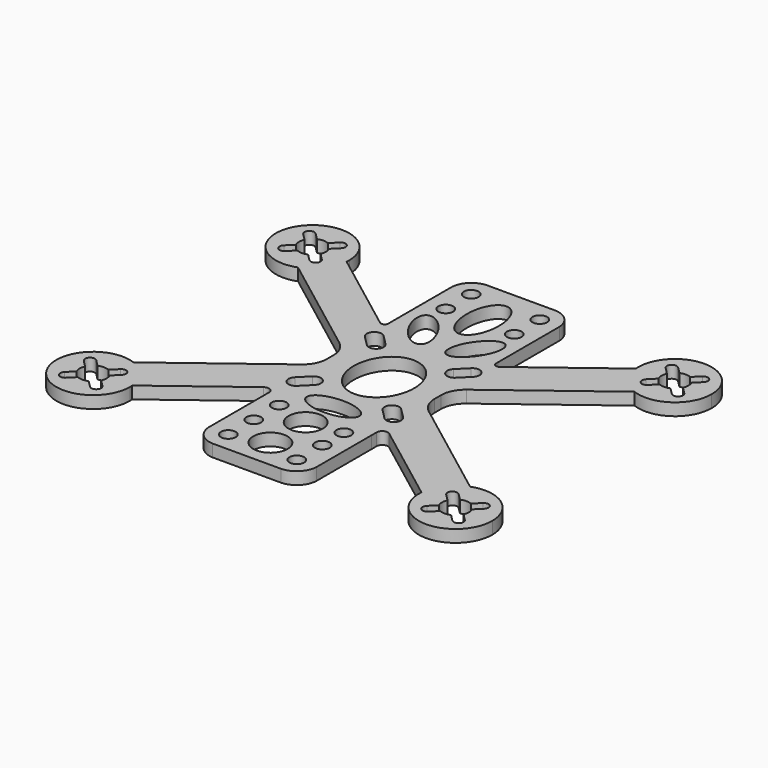
from build123d import *

# Parameters (mm, degrees)
F0_R     = 1.5
F0_R_2   = 3.5
F1_DEPTH = 2.5


# Not quite as in the source:
# - ends of sketch curves that miss each other by under 0.0002 mm in the source are joined


with BuildPart() as f1:
    # F0 (on Top) → F1 (new body)
    with BuildSketch(Plane.XY):
        with BuildLine():
            ThreePointArc((34.3547960707, 20.9819592355), (41.2667886361, 21.831976432), (44.5, 28))
            ThreePointArc((44.5, 28), (36.6803140057, 35.4931836268), (29.5272531026, 27.3612091045))
            ThreePointArc((29.5272531026, 27.3612091045), (31.0194532478, 23.4741784675), (34.3547960707, 20.9819592355))
        make_face()
        with BuildLine():
            ThreePointArc((39.5185288745, 29.1043153121), (39.6915102085, 28.5641567137), (39.75, 28))
            ThreePointArc((39.75, 28), (39.6915102085, 27.4358432863), (39.5185288745, 26.8956846879))
            Line((39.5185288745, 26.8956846879), (40.8890872965, 25.5251262658))
            ThreePointArc((40.8890872965, 25.5251262658), (41.1058600479, 25.200702917), (41.1819805153, 24.8180194847))
            ThreePointArc((41.1819805153, 24.8180194847), (40.5646639477, 23.8941399521), (39.4748737342, 24.1109127035))
            Line((39.4748737342, 24.1109127035), (38.1043153121, 25.4814711255))
            ThreePointArc((38.1043153121, 25.4814711255), (37, 25.25), (35.8956846879, 25.4814711255))
            Line((35.8956846879, 25.4814711255), (34.5251262658, 24.1109127035))
            ThreePointArc((34.5251262658, 24.1109127035), (33.1109127035, 24.1109127035), (33.1109127035, 25.5251262658))
            Line((33.1109127035, 25.5251262658), (34.4814711255, 26.8956846879))
            ThreePointArc((34.4814711255, 26.8956846879), (34.25, 28), (34.4814711255, 29.1043153121))
            Line((34.4814711255, 29.1043153121), (33.1109127035, 30.4748737342))
            ThreePointArc((33.1109127035, 30.4748737342), (33.1109127035, 31.8890872965), (34.5251262659, 31.8890872965))
            Line((34.5251262659, 31.8890872965), (35.8956846879, 30.5185288745))
            ThreePointArc((35.8956846879, 30.5185288745), (37, 30.75), (38.1043153121, 30.5185288745))
            Line((38.1043153121, 30.5185288745), (39.4748737342, 31.8890872965))
            ThreePointArc((39.4748737342, 31.8890872965), (40.5646639477, 32.1058600479), (41.1819805153, 31.1819805153))
            ThreePointArc((41.1819805153, 31.1819805153), (41.1058600479, 30.799297083), (40.8890872965, 30.4748737342))
            Line((40.8890872965, 30.4748737342), (39.5185288745, 29.1043153121))
        make_face(mode=Mode.SUBTRACT)
        with BuildLine():
            ThreePointArc((34.3547960707, 20.9819592355), (31.0194532478, 23.4741784675), (29.5272531026, 27.3612091045))
            Line((29.5272531026, 27.3612091045), (12.1863106506, 14.2383327238))
            ThreePointArc((12.1863106506, 14.2383327238), (11.4103948027, 14.1658389401), (10.9999810531, 14.8283050191))
            Line((10.9999810531, 14.8283050191), (10.9999810531, 15.3887438851))
            Line((10.9999810531, 15.3887438851), (11, 30.9999999999))
            ThreePointArc((11, 30.9999999999), (9.7793705992, 33.7793705992), (7, 35))
            Line((7, 35), (-7, 35))
            ThreePointArc((-7, 35), (-9.7793705992, 33.7793705992), (-11, 30.9999999999))
            Line((-11, 30.9999999999), (-11.0000189469, 15.3887625552))
            Line((-11.0000189469, 15.3887625552), (-11.0000085785, 14.8283395373))
            ThreePointArc((-11.0000085785, 14.8283395373), (-11.4104161998, 14.1658628176), (-12.1863381759, 14.2383535537))
            Line((-12.1863381759, 14.2383535537), (-29.5272531027, 27.3612091045))
            ThreePointArc((-29.5272531027, 27.3612091045), (-31.0194532478, 23.4741784675), (-34.3547960707, 20.9819592355))
            Line((-34.3547960707, 20.9819592355), (-12.9827933492, 4.8085505238))
            ThreePointArc((-12.9827933492, 4.8085505238), (-11.5230630838, 3.0479451115), (-11.0000068481, 0.8215228605))
            Line((-11.0000068481, 0.8215228605), (-11.0000054834, -0.8215135223))
            ThreePointArc((-11.0000054834, -0.8215135223), (-11.52305987, -3.0479403605), (-12.9827919846, -4.8085494911))
            Line((-12.9827919846, -4.8085494911), (-34.3547960707, -20.9819592355))
            ThreePointArc((-34.3547960707, -20.9819592355), (-31.0194532478, -23.4741784675), (-29.5272531026, -27.3612091045))
            Line((-29.5272531026, -27.3612091045), (-12.8232836871, -14.7203664102))
            ThreePointArc((-12.8232836871, -14.7203664102), (-11.6307646479, -14.6089516643), (-10.9999982035, -15.6271110806))
            Line((-10.9999982035, -15.6271110806), (-11.0000078854, -16.9179276686))
            Line((-11.0000078854, -16.9179276686), (-11, -30.9999999999))
            ThreePointArc((-11, -30.9999999999), (-9.7793705992, -33.7793705992), (-7, -35))
            Line((-7, -35), (7, -35))
            ThreePointArc((7, -35), (9.7793705992, -33.7793705992), (11, -30.9999999999))
            Line((11, -30.9999999999), (11.0000078854, -16.9179276686))
            Line((11.0000078854, -16.9179276686), (10.9999982035, -15.6271110806))
            ThreePointArc((10.9999982035, -15.6271110806), (11.6307646479, -14.6089516643), (12.8232836871, -14.7203664102))
            Line((12.8232836871, -14.7203664102), (29.5272531027, -27.3612091045))
            ThreePointArc((29.5272531027, -27.3612091045), (31.0194532478, -23.4741784675), (34.3547960707, -20.9819592355))
            Line((34.3547960707, -20.9819592355), (12.9827810177, -4.8085411919))
            ThreePointArc((12.9827810177, -4.8085411919), (11.5230507523, -3.0479357796), (10.9999945166, -0.8215135285))
            Line((10.9999945166, -0.8215135285), (10.999993152, 0.8215041904))
            ThreePointArc((10.999993152, 0.8215041904), (11.5230475385, 3.0479310286), (12.9827796531, 4.8085401592))
            Line((12.9827796531, 4.8085401592), (34.3547960707, 20.9819592355))
        make_face()
        with Locations((-7, -30.9999999999)):
            Circle(F0_R, mode=Mode.SUBTRACT)
        with Locations((-7, -24.4999999999)):
            Circle(F0_R, mode=Mode.SUBTRACT)
        with Locations((-7, -17.9999999999)):
            Circle(F0_R, mode=Mode.SUBTRACT)
        with BuildLine():
            ThreePointArc((-9.0606601718, -6.9393398282), (-7.4259748515, -6.6141807012), (-6.5, -8))
            ThreePointArc((-6.5, -8), (-6.6141807012, -8.5740251485), (-6.9393398282, -9.0606601717))
            Line((-6.9393398282, -9.0606601717), (-8.9393398282, -11.0606601717))
            ThreePointArc((-8.9393398282, -11.0606601717), (-11.0606601718, -11.0606601718), (-11.0606601718, -8.9393398282))
            Line((-11.0606601718, -8.9393398282), (-9.0606601718, -6.9393398282))
        make_face(mode=Mode.SUBTRACT)
        with Locations((0, -28.9999999999)):
            Circle(F0_R_2, mode=Mode.SUBTRACT)
        with Locations((7, -30.9999999999)):
            Circle(F0_R, mode=Mode.SUBTRACT)
        with Locations((7, -24.5)):
            Circle(F0_R, mode=Mode.SUBTRACT)
        with Locations((0, -19.9999999999)):
            Circle(F0_R_2, mode=Mode.SUBTRACT)
        with Locations((7, -19)):
            Circle(F0_R, mode=Mode.SUBTRACT)
        with BuildLine():
            add(Edge.make_bspline(
                [(5.3534731269, -12.9912551492), (5.3534731269, -8.6611281303), (-2.6767365634, -10.8261916398), (-10.7069462538, -12.9912551492), (-2.6767365634, -15.1563186587), (5.3534731269, -17.3213821682), (5.3534731269, -12.9912551492)],
                knots=[0, 0, 0, 2.0943951024, 2.0943951024, 4.1887902048, 4.1887902048, 6.2831853072, 6.2831853072, 6.2831853072], degree=2, weights=[1, 0.5, 1, 0.5, 1, 0.5, 1]))
        make_face(mode=Mode.SUBTRACT)
        with BuildLine():
            ThreePointArc((6.9393398282, -9.0606601717), (6.9393398282, -6.9393398282), (9.0606601718, -6.9393398282))
            Line((9.0606601718, -6.9393398282), (11.0606601718, -8.9393398282))
            ThreePointArc((11.0606601718, -8.9393398282), (11.3858192988, -9.4259748515), (11.5, -10))
            ThreePointArc((11.5, -10), (10.5740251485, -11.3858192988), (8.9393398282, -11.0606601717))
            Line((8.9393398282, -11.0606601717), (6.9393398282, -9.0606601717))
        make_face(mode=Mode.SUBTRACT)
        with BuildLine():
            ThreePointArc((-6.9393398282, 9.0606601717), (-6.6141807012, 8.5740251485), (-6.5, 8))
            ThreePointArc((-6.5, 8), (-7.4259748515, 6.6141807012), (-9.0606601718, 6.9393398282))
            Line((-9.0606601718, 6.9393398282), (-11.0606601718, 8.9393398282))
            ThreePointArc((-11.0606601718, 8.9393398282), (-11.0606601718, 11.0606601718), (-8.9393398282, 11.0606601717))
            Line((-8.9393398282, 11.0606601717), (-6.9393398282, 9.0606601717))
        make_face(mode=Mode.SUBTRACT)
        with BuildLine():
            add(Edge.make_bspline(
                [(-2.6455968618, 12.4099850655), (0.8605262478, 14.6258535456), (-4.929215171, 19.9050748086), (-10.7189565897, 25.1842960715), (-8.4353382806, 17.6892063284), (-6.1517199715, 10.1941165853), (-2.6455968618, 12.4099850655)],
                knots=[0, 0, 0, 2.0943951024, 2.0943951024, 4.1887902048, 4.1887902048, 6.2831853072, 6.2831853072, 6.2831853072], degree=2, weights=[1, 0.5, 1, 0.5, 1, 0.5, 1]))
        make_face(mode=Mode.SUBTRACT)
        with Locations((-7, 24.4999999999)):
            Circle(F0_R, mode=Mode.SUBTRACT)
        with Locations((-7, 30.9999999999)):
            Circle(F0_R, mode=Mode.SUBTRACT)
        with BuildLine():
            add(Edge.make_bspline(
                [(6.170543842, 0), (6.170543842, 12.9903810568), (-3.085271921, 6.4951905284), (-12.341087684, 0), (-3.085271921, -6.4951905284), (6.170543842, -12.9903810568), (6.170543842, 0)],
                knots=[4.7123889804, 4.7123889804, 4.7123889804, 6.8067840828, 6.8067840828, 8.9011791852, 8.9011791852, 10.9955742876, 10.9955742876, 10.9955742876], degree=2, weights=[1, 0.5, 1, 0.5, 1, 0.5, 1]))
        make_face(mode=Mode.SUBTRACT)
        with BuildLine():
            ThreePointArc((9.0606601718, 6.9393398282), (6.9393398282, 6.9393398282), (6.9393398282, 9.0606601717))
            Line((6.9393398282, 9.0606601717), (8.9393398282, 11.0606601717))
            ThreePointArc((8.9393398282, 11.0606601717), (10.5740251485, 11.3858192988), (11.5, 10))
            ThreePointArc((11.5, 10), (11.3858192988, 9.4259748515), (11.0606601718, 8.9393398282))
            Line((11.0606601718, 8.9393398282), (9.0606601718, 6.9393398282))
        make_face(mode=Mode.SUBTRACT)
        with BuildLine():
            add(Edge.make_bspline(
                [(2.6455968618, 12.4099850655), (6.1517199715, 10.1941165853), (8.4353382806, 17.6892063284), (10.7189565897, 25.1842960715), (4.929215171, 19.9050748086), (-0.8605262478, 14.6258535456), (2.6455968618, 12.4099850655)],
                knots=[0, 0, 0, 2.0943951024, 2.0943951024, 4.1887902048, 4.1887902048, 6.2831853072, 6.2831853072, 6.2831853072], degree=2, weights=[1, 0.5, 1, 0.5, 1, 0.5, 1]))
        make_face(mode=Mode.SUBTRACT)
        with BuildLine():
            add(Edge.make_bspline(
                [(0, 19.1709659993), (5.6914834307, 19.1709659993), (2.8457417153, 28.2382629811), (0, 37.3055599629), (-2.8457417153, 28.2382629811), (-5.6914834307, 19.1709659993), (0, 19.1709659993)],
                knots=[0, 0, 0, 2.0943951024, 2.0943951024, 4.1887902048, 4.1887902048, 6.2831853072, 6.2831853072, 6.2831853072], degree=2, weights=[1, 0.5, 1, 0.5, 1, 0.5, 1]))
        make_face(mode=Mode.SUBTRACT)
        with Locations((7, 24.5)):
            Circle(F0_R, mode=Mode.SUBTRACT)
        with Locations((7, 30.9999999999)):
            Circle(F0_R, mode=Mode.SUBTRACT)
        with BuildLine():
            ThreePointArc((44.5, -28), (41.2667886361, -21.831976432), (34.3547960707, -20.9819592355))
            ThreePointArc((34.3547960707, -20.9819592355), (31.0194532478, -23.4741784675), (29.5272531026, -27.3612091045))
            ThreePointArc((29.5272531026, -27.3612091045), (36.6803140057, -35.4931836268), (44.5, -28))
        make_face()
        with BuildLine():
            ThreePointArc((39.5185288745, -26.8956846879), (39.6915102085, -27.4358432863), (39.75, -28))
            ThreePointArc((39.75, -28), (39.6915102085, -28.5641567137), (39.5185288745, -29.1043153121))
            Line((39.5185288745, -29.1043153121), (40.8890872965, -30.4748737342))
            ThreePointArc((40.8890872965, -30.4748737342), (41.1058600479, -30.799297083), (41.1819805153, -31.1819805153))
            ThreePointArc((41.1819805153, -31.1819805153), (40.5646639477, -32.1058600479), (39.4748737342, -31.8890872965))
            Line((39.4748737342, -31.8890872965), (38.1043153121, -30.5185288745))
            ThreePointArc((38.1043153121, -30.5185288745), (37, -30.75), (35.8956846879, -30.5185288745))
            Line((35.8956846879, -30.5185288745), (34.5251262659, -31.8890872965))
            ThreePointArc((34.5251262659, -31.8890872965), (33.1109127035, -31.8890872965), (33.1109127035, -30.4748737342))
            Line((33.1109127035, -30.4748737342), (34.4814711255, -29.1043153121))
            ThreePointArc((34.4814711255, -29.1043153121), (34.25, -28), (34.4814711255, -26.8956846879))
            Line((34.4814711255, -26.8956846879), (33.1109127035, -25.5251262658))
            ThreePointArc((33.1109127035, -25.5251262658), (33.1109127035, -24.1109127035), (34.5251262658, -24.1109127035))
            Line((34.5251262658, -24.1109127035), (35.8956846879, -25.4814711255))
            ThreePointArc((35.8956846879, -25.4814711255), (37, -25.25), (38.1043153121, -25.4814711255))
            Line((38.1043153121, -25.4814711255), (39.4748737342, -24.1109127035))
            ThreePointArc((39.4748737342, -24.1109127035), (40.5646639477, -23.8941399521), (41.1819805153, -24.8180194847))
            ThreePointArc((41.1819805153, -24.8180194847), (41.1058600479, -25.200702917), (40.8890872965, -25.5251262658))
            Line((40.8890872965, -25.5251262658), (39.5185288745, -26.8956846879))
        make_face(mode=Mode.SUBTRACT)
        with BuildLine():
            ThreePointArc((-34.3547960707, 20.9819592355), (-31.0194532478, 23.4741784675), (-29.5272531026, 27.3612091045))
            ThreePointArc((-29.5272531026, 27.3612091045), (-29.5068163732, 27.6803140057), (-29.5, 28))
            ThreePointArc((-29.5, 28), (-43.168023568, 32.2667886361), (-34.3547960707, 20.9819592355))
        make_face()
        with BuildLine():
            ThreePointArc((-34.4814711255, 29.1043153121), (-34.3084897915, 28.5641567137), (-34.25, 28))
            ThreePointArc((-34.25, 28), (-34.3084897915, 27.4358432863), (-34.4814711255, 26.8956846879))
            Line((-34.4814711255, 26.8956846879), (-33.1109127035, 25.5251262658))
            ThreePointArc((-33.1109127035, 25.5251262658), (-32.8941399521, 25.200702917), (-32.8180194847, 24.8180194847))
            ThreePointArc((-32.8180194847, 24.8180194847), (-33.4353360523, 23.8941399521), (-34.5251262658, 24.1109127035))
            Line((-34.5251262658, 24.1109127035), (-35.8956846879, 25.4814711255))
            ThreePointArc((-35.8956846879, 25.4814711255), (-37, 25.25), (-38.1043153121, 25.4814711255))
            Line((-38.1043153121, 25.4814711255), (-39.4748737342, 24.1109127035))
            ThreePointArc((-39.4748737342, 24.1109127035), (-40.8890872965, 24.1109127035), (-40.8890872965, 25.5251262658))
            Line((-40.8890872965, 25.5251262658), (-39.5185288745, 26.8956846879))
            ThreePointArc((-39.5185288745, 26.8956846879), (-39.75, 28), (-39.5185288745, 29.1043153121))
            Line((-39.5185288745, 29.1043153121), (-40.8890872965, 30.4748737342))
            ThreePointArc((-40.8890872965, 30.4748737342), (-40.8890872965, 31.8890872965), (-39.4748737342, 31.8890872965))
            Line((-39.4748737342, 31.8890872965), (-38.1043153121, 30.5185288745))
            ThreePointArc((-38.1043153121, 30.5185288745), (-37, 30.75), (-35.8956846879, 30.5185288745))
            Line((-35.8956846879, 30.5185288745), (-34.5251262659, 31.8890872965))
            ThreePointArc((-34.5251262659, 31.8890872965), (-33.4353360523, 32.1058600479), (-32.8180194847, 31.1819805153))
            ThreePointArc((-32.8180194847, 31.1819805153), (-32.8941399522, 30.799297083), (-33.1109127035, 30.4748737342))
            Line((-33.1109127035, 30.4748737342), (-34.4814711255, 29.1043153121))
        make_face(mode=Mode.SUBTRACT)
        with BuildLine():
            ThreePointArc((-29.5272531026, -27.3612091045), (-31.0194532478, -23.4741784675), (-34.3547960707, -20.9819592355))
            ThreePointArc((-34.3547960707, -20.9819592355), (-43.168023568, -32.2667886361), (-29.5, -28))
            ThreePointArc((-29.5, -28), (-29.5068163732, -27.6803140057), (-29.5272531026, -27.3612091045))
        make_face()
        with BuildLine():
            ThreePointArc((-34.4814711255, -26.8956846879), (-34.3084897915, -27.4358432863), (-34.25, -28))
            ThreePointArc((-34.25, -28), (-34.3084897915, -28.5641567137), (-34.4814711255, -29.1043153121))
            Line((-34.4814711255, -29.1043153121), (-33.1109127035, -30.4748737342))
            ThreePointArc((-33.1109127035, -30.4748737342), (-32.8941399522, -30.799297083), (-32.8180194847, -31.1819805153))
            ThreePointArc((-32.8180194847, -31.1819805153), (-33.4353360523, -32.1058600479), (-34.5251262659, -31.8890872965))
            Line((-34.5251262659, -31.8890872965), (-35.8956846879, -30.5185288745))
            ThreePointArc((-35.8956846879, -30.5185288745), (-37, -30.75), (-38.1043153121, -30.5185288745))
            Line((-38.1043153121, -30.5185288745), (-39.4748737342, -31.8890872965))
            ThreePointArc((-39.4748737342, -31.8890872965), (-40.8890872965, -31.8890872965), (-40.8890872965, -30.4748737342))
            Line((-40.8890872965, -30.4748737342), (-39.5185288745, -29.1043153121))
            ThreePointArc((-39.5185288745, -29.1043153121), (-39.75, -28), (-39.5185288745, -26.8956846879))
            Line((-39.5185288745, -26.8956846879), (-40.8890872965, -25.5251262658))
            ThreePointArc((-40.8890872965, -25.5251262658), (-40.8890872965, -24.1109127035), (-39.4748737342, -24.1109127035))
            Line((-39.4748737342, -24.1109127035), (-38.1043153121, -25.4814711255))
            ThreePointArc((-38.1043153121, -25.4814711255), (-37, -25.25), (-35.8956846879, -25.4814711255))
            Line((-35.8956846879, -25.4814711255), (-34.5251262658, -24.1109127035))
            ThreePointArc((-34.5251262658, -24.1109127035), (-33.4353360523, -23.8941399521), (-32.8180194847, -24.8180194847))
            ThreePointArc((-32.8180194847, -24.8180194847), (-32.8941399521, -25.200702917), (-33.1109127035, -25.5251262658))
            Line((-33.1109127035, -25.5251262658), (-34.4814711255, -26.8956846879))
        make_face(mode=Mode.SUBTRACT)
    extrude(amount=F1_DEPTH)


solid = f1.part
